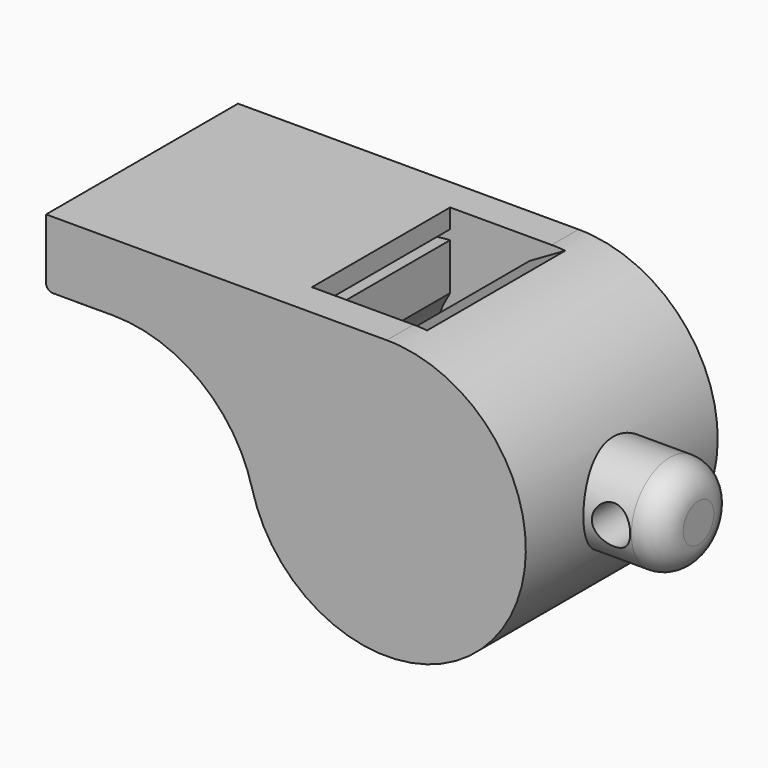
from build123d import *

# Parameters (mm, degrees)
F0_W          = 24.9102279718
F0_H          = 2
F1_DEPTH      = 12.5
F2_DEPTH      = 9
F5_W          = 10
F5_H          = 5
F7_R          = 3
F8_R          = 2
F9_DEPTH      = 12.5010001
F9_DEPTH_BACK = 12.5010001
F10_W         = 4
F10_H         = 20
F11_DEPTH     = 2
F12_F1_R      = 0.7
F12_F2_R      = 0.7
F12_F3_R      = 0.7
F12_F4_R      = 0.7
F12_F5_R      = 0.7
F13_R         = 15


with BuildPart() as f1:
    # F0 (on Front) → F1 (new body, symmetric)
    with BuildSketch(Plane.XZ):
        with BuildLine():
            Line((-10.5897720282, 11.5), (-35.5, 9))
            Line((-35.5, 9), (-35.5, 7.5))
            Line((-35.5, 7.5), (-12.409673646, 7.5))
            ThreePointArc((-12.409673646, 7.5), (6.5005800977, -12.9611904698), (1.4102279718, 14.4312597187))
            Line((1.4102279718, 14.4312597187), (-2.3066189308, 12.2853371589))
            ThreePointArc((-2.3066189308, 12.2853371589), (7.0386819061, -10.3299059543), (-10.5897720282, 6.6412896632))
            Line((-10.5897720282, 6.6412896632), (-10.5897720282, 11.5))
        make_face()
        with Locations((-23.0448860141, 13.5)):
            Rectangle(F0_W, F0_H)
        with BuildLine():
            Line((-35.5, 12.5), (-35.5, 9))
            Line((-35.5, 9), (-10.5897720282, 11.5))
            Line((-10.5897720282, 11.5), (-10.5897720282, 6.6412896632))
            ThreePointArc((-10.5897720282, 6.6412896632), (7.0386819061, -10.3299059543), (-2.3066189308, 12.2853371589))
            Line((-2.3066189308, 12.2853371589), (1.4102279718, 14.4312597187))
            ThreePointArc((1.4102279718, 14.4312597187), (0.7059511596, 14.4828047339), (0, 14.5))
            Line((0, 14.5), (-10.5897720282, 14.5))
            Line((-10.5897720282, 14.5), (-10.5897720282, 12.5))
            Line((-10.5897720282, 12.5), (-35.5, 12.5))
        make_face()
    extrude(amount=F1_DEPTH, both=True)

    # F0 (on Front) → F2 (cut, symmetric)
    with BuildSketch(Plane.XZ):
        with BuildLine():
            Line((-35.5, 12.5), (-35.5, 9))
            Line((-35.5, 9), (-10.5897720282, 11.5))
            Line((-10.5897720282, 11.5), (-10.5897720282, 6.6412896632))
            ThreePointArc((-10.5897720282, 6.6412896632), (7.0386819061, -10.3299059543), (-2.3066189308, 12.2853371589))
            Line((-2.3066189308, 12.2853371589), (1.4102279718, 14.4312597187))
            ThreePointArc((1.4102279718, 14.4312597187), (0.7059511596, 14.4828047339), (0, 14.5))
            Line((0, 14.5), (-10.5897720282, 14.5))
            Line((-10.5897720282, 14.5), (-10.5897720282, 12.5))
            Line((-10.5897720282, 12.5), (-35.5, 12.5))
        make_face()
    extrude(amount=F2_DEPTH, both=True, mode=Mode.SUBTRACT)

    # F5 (on Front) → F6 (revolve)
    with BuildSketch(Plane.XZ):
        with Locations((17.5, 2.5)):
            Rectangle(F5_W, F5_H)
    revolve(axis=Axis((17.5, 0, 0), (1, 0, 0)))

    # F7
    f7_edges = [f1.edges().sort_by_distance(p)[0] for p in [
        (22.5, 0, -5),
    ]]
    fillet(f7_edges, radius=F7_R)

    # F8 (on Front) → F9 (cut, two sides)
    with BuildSketch(Plane.XZ) as f9_sk:
        with Locations((17.38, 0)):
            Circle(F8_R)
    extrude(amount=F9_DEPTH, mode=Mode.SUBTRACT)
    extrude(f9_sk.sketch, amount=-F9_DEPTH_BACK, mode=Mode.SUBTRACT)

    # F10 (on face) → F11 (join)
    with BuildSketch(Plane(origin=(0, 0, 7.5), x_dir=(1, 0, 0), z_dir=(0, 0, -1))):
        with Locations((-33.5, 0)):
            Rectangle(F10_W, F10_H)
    extrude(amount=F11_DEPTH)

    # F12: fillet of radius 0.7 on 11 edges, made by hand

    # F12_f1
    f12_f1_edges = [f1.edges().sort_by_distance(p)[0] for p in [
        (-31.5, 10, 6.5),
    ]]
    fillet(f12_f1_edges, radius=F12_F1_R)

    # F12_f2
    f12_f2_edges = [f1.edges().sort_by_distance(p)[0] for p in [
        (-31.5, -10, 6.5),
    ]]
    fillet(f12_f2_edges, radius=F12_F2_R)

    # F12_f3
    f12_f3_edges = [f1.edges().sort_by_distance(p)[0] for p in [
        (-33.85, 10, 7.5),
    ]]
    fillet(f12_f3_edges, radius=F12_F3_R)

    # F12_f4
    f12_f4_edges = [f1.edges().sort_by_distance(p)[0] for p in [
        (-33.85, 10, 5.5),
    ]]
    fillet(f12_f4_edges, radius=F12_F4_R)

    # F12_f5
    f12_f5_edges = [f1.edges().sort_by_distance(p)[0] for p in [
        (-35.5, 0, 5.5),
    ]]
    fillet(f12_f5_edges, radius=F12_F5_R)

    # F13
    f13_edges = [f1.edges().sort_by_distance(p)[0] for p in [
        (-12.409674, 0, 7.5),
    ]]
    fillet(f13_edges, radius=F13_R)


with BuildPart() as f4:
    # F3 (on Front) → F4 (revolve)
    with BuildSketch(Plane.XZ):
        with BuildLine():
            Line((0, -12), (0, -1))
            ThreePointArc((0, -1), (-5.5, -6.5), (0, -12))
        make_face()
    revolve(axis=Axis((0, 0, -6.5), (0, 0, -1)))


solid = Compound([f1.part, f4.part])
